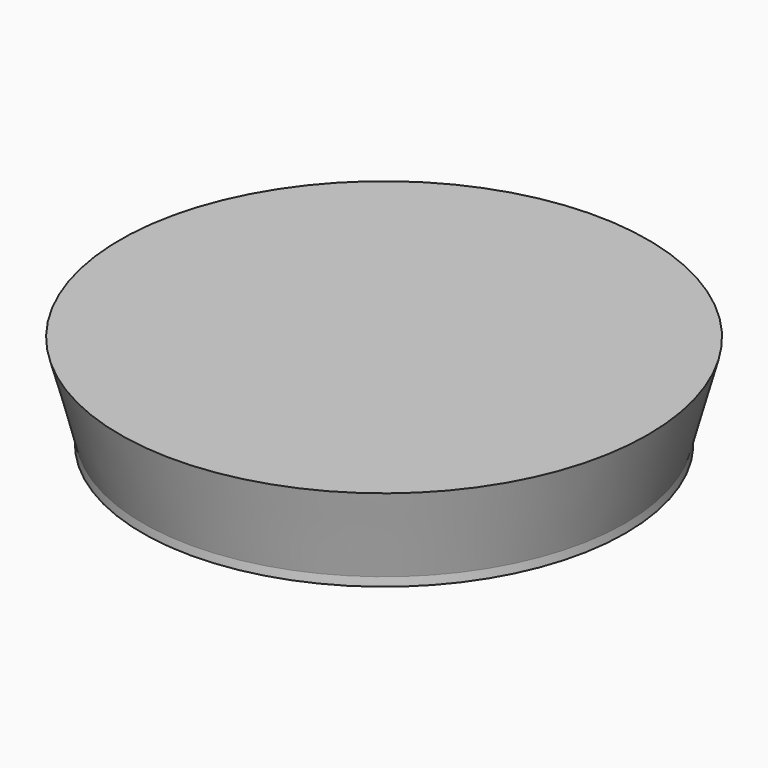
from build123d import *

# Parameters (mm, degrees)
F0_R          = 70.5568902051
F1_DEPTH      = 25
F1_TAPER      = -15
F1_DEPTH_BACK = 2.5
F1_TAPER_BACK = -3


with BuildPart() as f1:
    # F0 (on Top) → F1 (new body, two sides)
    with BuildSketch(Plane.XY) as f1_sk:
        Circle(F0_R)
    extrude(amount=F1_DEPTH, taper=F1_TAPER)
    extrude(f1_sk.sketch, amount=-F1_DEPTH_BACK, taper=F1_TAPER_BACK)


solid = f1.part
